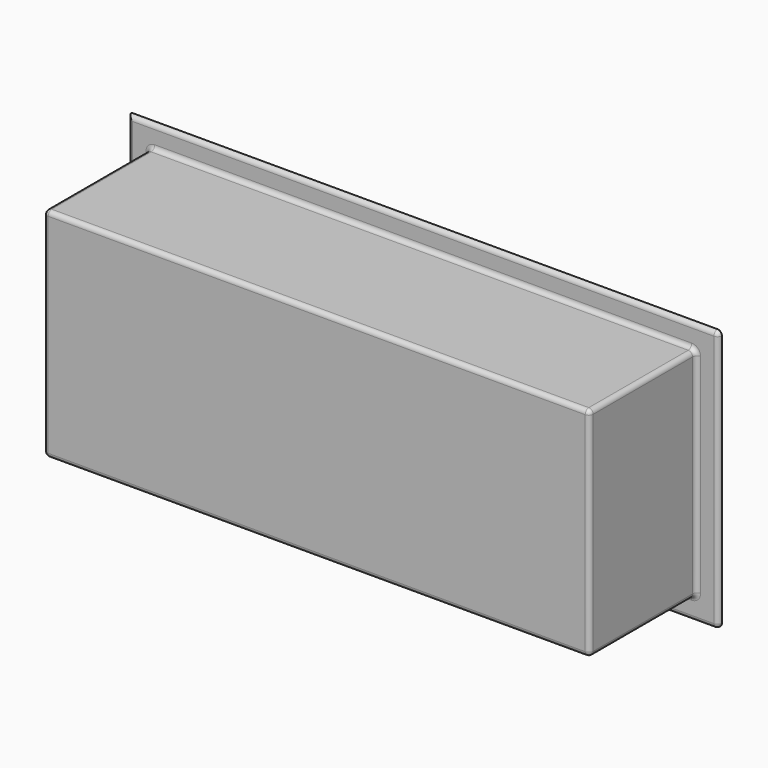
from build123d import *

# Parameters (mm, degrees)
F1_W        = 123
F1_H        = 49
F1_W_2      = 119
F1_H_2      = 45
F2_DEPTH    = 31
F1_H_3      = 5
F3_DEPTH    = 1
F4_DEPTH    = 31
F5_DEPTH    = 29
F6_F1_R     = 0.9999
F6_F2_R     = 1
F7_T1_DEPTH = 3.5
F7_T4_ANGLE = 90
F7_T6_ANGLE = 90
F7_T8_ANGLE = 90


# Not quite as in the source:
# - a fillet or chamfer that OpenCascade refuses, or shapes differently, is made with other operations: its cross-section is extruded or revolved along the edge and cut away or added
# - a fillet or chamfer is up to 0.001 mm smaller than in the source, because OpenCascade refuses the exact size


with BuildPart() as f2:
    # F1 (on offset) → F2 (new body)
    with BuildSketch(Plane.XZ.offset(15)):
        Rectangle(F1_W, F1_H)
        Rectangle(F1_W_2, F1_H_2, mode=Mode.SUBTRACT)
    extrude(amount=F2_DEPTH)

    # F1 (on offset) → F3 (join)
    with BuildSketch(Plane.XZ.offset(15)):
        with Locations((0, 27)):
            Rectangle(F1_W, F1_H_3)
        Polygon((-61.5, -29.5), (-61.5, -24.5), (-61.5, 24.5), (-61.5, 29.5), (-66.5, 29.5), (-66.5, -29.5), align=None)
        with Locations((0, -27)):
            Rectangle(F1_W, F1_H_3)
        Polygon((61.5, 24.5), (61.5, -24.5), (61.5, -29.5), (66.5, -29.5), (66.5, 29.5), (61.5, 29.5), align=None)
    extrude(amount=F3_DEPTH)

    # F1 (on offset) → F4 (join)
    with BuildSketch(Plane.XZ.offset(15)):
        Rectangle(F1_W_2, F1_H_2)
    extrude(amount=F4_DEPTH)

    # F1 (on offset) → F5 (cut)
    with BuildSketch(Plane.XZ.offset(15)):
        Rectangle(F1_W_2, F1_H_2)
    extrude(amount=F5_DEPTH, mode=Mode.SUBTRACT)

    # F6: fillet of radius 1 on 14 edges, made by hand

    # F6_f1 (radius 1 in the source; OpenCascade refuses exactly that, so slightly less here)
    f6_f1_edges = [f2.edges().sort_by_distance(p)[0] for p in [
        (61.5, -31, 24.5),
        (61.5, -31, -24.5),
        (61.5, -46, 0),
        (0, -46, -24.5),
        (0, -46, 24.5),
        (-61.5, -31, -24.5),
        (-61.5, -31, 24.5),
        (-61.5, -46, 0),
        (0, -16, -29.5),
        (-66.5, -16, 0),
        (0, -16, 29.5),
        (66.5, -16, 0),
    ]]
    fillet(f6_f1_edges, radius=F6_F1_R)

    # F6_f2
    f6_f2_edges = [f2.edges().sort_by_distance(p)[0] for p in [
        (61.5, -16, 0),
        (-61.5, -16, 0),
        (-61.2071360705, -16, -24.2071360705),
        (-61.2071360705, -16, 24.2071360705),
        (61.2071360705, -16, 24.2071360705),
        (61.2071360705, -16, -24.2071360705),
    ]]
    fillet(f6_f2_edges, radius=F6_F2_R)

    # F7: fillet of radius 1 on 7 edges, made by hand

    # F7_s2 → F7_t1 (cut)
    with BuildSketch(Plane.XZ.offset(12.5)):
        with BuildLine():
            ThreePointArc((-65.5, -29.5), (-66.2071067812, -29.2071067812), (-66.5, -28.5))
            Line((-66.5, -28.5), (-66.5, -29.5))
            Line((-66.5, -29.5), (-65.5, -29.5))
        make_face()
        with BuildLine():
            ThreePointArc((65.5, -29.5), (66.2071067812, -29.2071067812), (66.5, -28.5))
            Line((66.5, -28.5), (66.5, -29.5))
            Line((66.5, -29.5), (65.5, -29.5))
        make_face()
        with BuildLine():
            ThreePointArc((66.5, 28.5), (66.2071067812, 29.2071067812), (65.5, 29.5))
            Line((65.5, 29.5), (66.5, 29.5))
            Line((66.5, 29.5), (66.5, 28.5))
        make_face()
    extrude(amount=F7_T1_DEPTH, mode=Mode.SUBTRACT)

    # F7_s3 → F7_t4 (revolve, cut)
    with BuildSketch(Plane.XY.offset(-28.5)):
        with BuildLine():
            ThreePointArc((-65.5001, -16), (-66.2071360705, -15.7071360705), (-66.5, -15.0001))
            Line((-66.5, -15.0001), (-66.5, -16))
            Line((-66.5, -16), (-65.5001, -16))
        make_face()
    revolve(axis=Axis((-65.5, -16, -28.5), (0, -1, 0)), revolution_arc=F7_T4_ANGLE, mode=Mode.SUBTRACT)

    # F7_s5 → F7_t6 (revolve, cut)
    with BuildSketch(Plane.YZ.offset(65.5)):
        with BuildLine():
            ThreePointArc((-16, -28.5001), (-15.7071360705, -29.2071360705), (-15.0001, -29.5))
            Line((-15.0001, -29.5), (-16, -29.5))
            Line((-16, -29.5), (-16, -28.5001))
        make_face()
    revolve(axis=Axis((65.5, -16, -28.5), (0, -1, 0)), revolution_arc=F7_T6_ANGLE, mode=Mode.SUBTRACT)

    # F7_s7 → F7_t8 (revolve, cut)
    with BuildSketch(Plane.XY.offset(28.5)):
        with BuildLine():
            ThreePointArc((65.5001, -16), (66.2071360705, -15.7071360705), (66.5, -15.0001))
            Line((66.5, -15.0001), (66.5, -16))
            Line((66.5, -16), (65.5001, -16))
        make_face()
    revolve(axis=Axis((65.5, -16, 28.5), (0, -1, 0)), revolution_arc=F7_T8_ANGLE, mode=Mode.SUBTRACT)


solid = f2.part
